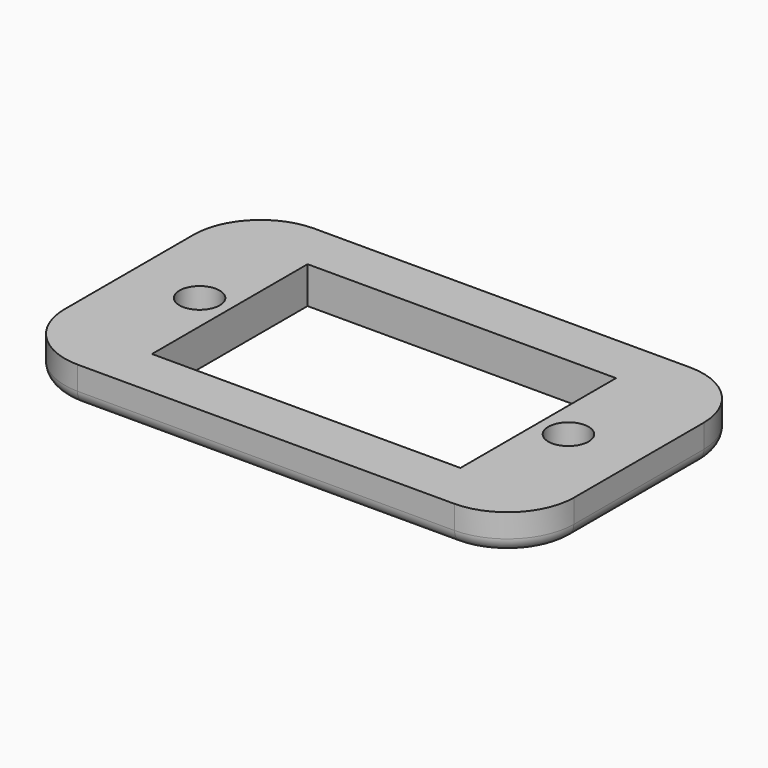
from build123d import *

# Parameters (mm, degrees)
F0_W         = 38
F0_H         = 22
F0_R         = 1.5
F0_W_2       = 23
F0_H_2       = 14.5
F1_DEPTH     = 2.75
F2_R         = 1
F3_T3_ANGLE  = 90
F3_T6_ANGLE  = 90
F3_T9_ANGLE  = 90
F3_T12_ANGLE = 90
F3_T15_DEPTH = 15.2524142536
F3_T18_DEPTH = 15.2524142536
F3_T21_DEPTH = 15.2524142536
F3_T24_DEPTH = 15.2524142536


# Not quite as in the source:
# - a fillet or chamfer that OpenCascade refuses, or shapes differently, is made with other operations: its cross-section is extruded or revolved along the edge and cut away or added


with BuildPart() as f1:
    # F0 (on Top) → F1 (new body)
    with BuildSketch(Plane.XY):
        with Locations((0.1353118792, -1.2320824713)):
            Rectangle(F0_W, F0_H)
        with Locations((-13.6146881208, -1.2320824713)):
            Circle(F0_R, mode=Mode.SUBTRACT)
        with Locations((0.1353118792, -1.2320824713)):
            Rectangle(F0_W_2, F0_H_2, mode=Mode.SUBTRACT)
        with Locations((13.8853118792, -1.2320824713)):
            Circle(F0_R, mode=Mode.SUBTRACT)
    extrude(amount=F1_DEPTH)

    # F2
    f2_edges = [f1.edges().sort_by_distance(p)[0] for p in [
        (19.135312, -1.232082, 0),
        (0.135312, 9.767918, 0),
        (-18.864688, -1.232082, 0),
        (0.135312, -12.232082, 0),
    ]]
    fillet(f2_edges, radius=F2_R)

    # F3: fillet of radius 5 on 4 edges, made by hand


with BuildPart() as f3_tool1:
    # F3_s2 → F3_t3 (revolve)
    with BuildSketch(Plane.XZ.offset(-4.7669518433)):
        with BuildLine():
            ThreePointArc((-17.8650881208, 0), (-18.572194902, 0.2928932188), (-18.8650881208, 1))
            Line((-18.8650881208, 1), (-18.8650881208, 0))
            Line((-18.8650881208, 0), (-17.8650881208, 0))
        make_face()
    revolve(axis=Axis((-13.8637224354, 4.7669518433, 0), (0, 0, -1)), revolution_arc=F3_T3_ANGLE)


with BuildPart() as f3_tool4:
    # F3_s5 → F3_t6 (revolve)
    with BuildSketch(Plane.YZ.offset(-13.8637224354)):
        with BuildLine():
            ThreePointArc((-11.2324824713, 0), (-11.9395892524, 0.2928932188), (-12.2324824713, 1))
            Line((-12.2324824713, 1), (-12.2324824713, 0))
            Line((-12.2324824713, 0), (-11.2324824713, 0))
        make_face()
    revolve(axis=Axis((-13.8637224354, -7.2311167858, 0), (0, 0, -1)), revolution_arc=F3_T6_ANGLE)


with BuildPart() as f3_tool7:
    # F3_s8 → F3_t9 (revolve)
    with BuildSketch(Plane.XZ.offset(7.2311167858)):
        with BuildLine():
            ThreePointArc((18.1357118792, 0), (18.8428186604, 0.2928932188), (19.1357118792, 1))
            Line((19.1357118792, 1), (19.1357118792, 0))
            Line((19.1357118792, 0), (18.1357118792, 0))
        make_face()
    revolve(axis=Axis((14.1343461938, -7.2311167858, 0), (0, 0, -1)), revolution_arc=F3_T9_ANGLE)


with BuildPart() as f3_tool10:
    # F3_s11 → F3_t12 (revolve)
    with BuildSketch(Plane.YZ.offset(14.1343461938)):
        with BuildLine():
            ThreePointArc((8.7683175287, 0), (9.4754243099, 0.2928932188), (9.7683175287, 1))
            Line((9.7683175287, 1), (9.7683175287, 0))
            Line((9.7683175287, 0), (8.7683175287, 0))
        make_face()
    revolve(axis=Axis((14.1343461938, 4.7669518433, 0), (0, 0, -1)), revolution_arc=F3_T12_ANGLE)


with BuildPart() as f3_tool13:
    # F3_s14 → F3_t15 (new body)
    with BuildSketch(Plane.XY):
        with BuildLine():
            ThreePointArc((14.1343461938, 9.7683175287), (17.6708457852, 8.3034514347), (19.1357118792, 4.7669518433))
            Line((19.1357118792, 4.7669518433), (19.6358484478, 4.7669518433))
            ThreePointArc((19.6358484478, 4.7669518433), (19.6354484478, 7.267434686), (19.6354484478, 9.7679175287))
            Line((19.6354484478, 9.7679175287), (19.1353118792, 10.2680540973))
            ThreePointArc((19.1353118792, 10.2680540973), (16.6348290365, 10.2680540973), (14.1343461938, 10.2684540973))
            Line((14.1343461938, 10.2684540973), (14.1343461938, 9.7683175287))
        make_face()
    extrude(amount=F3_T15_DEPTH)


with BuildPart() as f3_tool16:
    # F3_s17 → F3_t18 (new body)
    with BuildSketch(Plane.XY):
        with BuildLine():
            ThreePointArc((19.1357118792, -7.2311167858), (17.6708457852, -10.7676163772), (14.1343461938, -12.2324824713))
            Line((14.1343461938, -12.2324824713), (14.1343461938, -12.7326190398))
            ThreePointArc((14.1343461938, -12.7326190398), (16.6348290365, -12.7322190398), (19.1353118792, -12.7322190398))
            Line((19.1353118792, -12.7322190398), (19.6354484478, -12.2320824713))
            ThreePointArc((19.6354484478, -12.2320824713), (19.6354484478, -9.7315996285), (19.6358484478, -7.2311167858))
            Line((19.6358484478, -7.2311167858), (19.1357118792, -7.2311167858))
        make_face()
    extrude(amount=F3_T18_DEPTH)


with BuildPart() as f3_tool19:
    # F3_s20 → F3_t21 (new body)
    with BuildSketch(Plane.XY):
        with BuildLine():
            ThreePointArc((-18.8650881208, -7.2311167858), (-17.4002220267, -10.7676163772), (-13.8637224354, -12.2324824713))
            Line((-13.8637224354, -12.2324824713), (-13.8637224354, -12.7326190398))
            ThreePointArc((-13.8637224354, -12.7326190398), (-16.3642052781, -12.7322190398), (-18.8646881208, -12.7322190398))
            Line((-18.8646881208, -12.7322190398), (-19.3648246893, -12.2320824713))
            ThreePointArc((-19.3648246893, -12.2320824713), (-19.3648246893, -9.7315996285), (-19.3652246893, -7.2311167858))
            Line((-19.3652246893, -7.2311167858), (-18.8650881208, -7.2311167858))
        make_face()
    extrude(amount=F3_T21_DEPTH)


with BuildPart() as f3_tool22:
    # F3_s23 → F3_t24 (new body)
    with BuildSketch(Plane.XY):
        with BuildLine():
            ThreePointArc((-13.8637224354, 9.7683175287), (-17.4002220267, 8.3034514347), (-18.8650881208, 4.7669518433))
            Line((-18.8650881208, 4.7669518433), (-19.3652246893, 4.7669518433))
            ThreePointArc((-19.3652246893, 4.7669518433), (-19.3648246893, 7.267434686), (-19.3648246893, 9.7679175287))
            Line((-19.3648246893, 9.7679175287), (-18.8646881208, 10.2680540973))
            ThreePointArc((-18.8646881208, 10.2680540973), (-16.3642052781, 10.2680540973), (-13.8637224354, 10.2684540973))
            Line((-13.8637224354, 10.2684540973), (-13.8637224354, 9.7683175287))
        make_face()
    extrude(amount=F3_T24_DEPTH)


with BuildPart() as f1_1:
    add(f1.part)

    # F3_t25: cut F3_tool1, F3_tool4, F3_tool7, F3_tool10, F3_tool13, F3_tool16, F3_tool19, F3_tool22
    add([f3_tool1.part, f3_tool4.part, f3_tool7.part, f3_tool10.part, f3_tool13.part, f3_tool16.part, f3_tool19.part, f3_tool22.part], mode=Mode.SUBTRACT)


solid = f1_1.part
